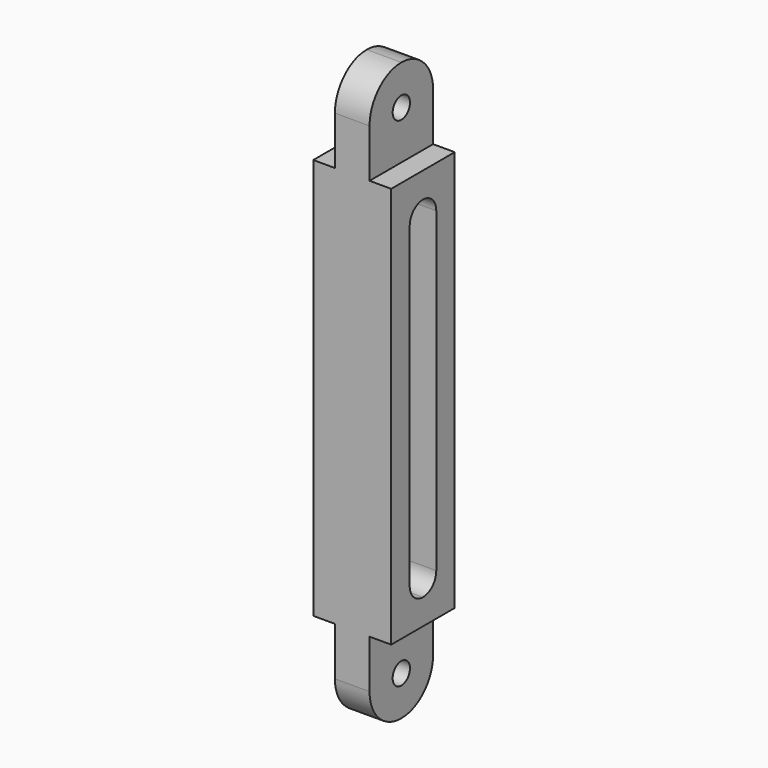
from build123d import *

# Parameters (mm, degrees)
F0_W      = 5.4
F0_H      = 40
F1_DEPTH  = 5.5
F2_W      = 1.5
F2_H      = 6.1
F3_DEPTH  = 5.501
F4_W      = 1.5
F4_H      = 6.1
F5_DEPTH  = 25
F6_W      = 1.5
F6_H      = 6.1
F7_DEPTH  = 5.501
F8_W      = 1.5
F8_H      = 6.1
F9_DEPTH  = 5.501
F10_R     = 2.75
F11_R     = 2.74999
F12_R     = 2.75
F13_R     = 2.74999
F14_W     = 2.3
F14_H     = 24.25
F15_DEPTH = 2.701
F16_DEPTH = 2.701
F17_R     = 1.15
F18_R     = 1.14999
F19_R     = 1.15
F20_R     = 1.14999
F21_R     = 0.75
F22_DEPTH = 3.901
F23_R     = 0.75
F24_DEPTH = 3.901


# Not quite as in the source:
# - a fillet or chamfer is up to 0.001 mm smaller than in the source, because OpenCascade refuses the exact size


with BuildPart() as f1:
    # F0 (on Front) → F1 (new body)
    with BuildSketch(Plane.XZ):
        Rectangle(F0_W, F0_H)
    extrude(amount=F1_DEPTH)

    # F2 (on face) → F3 (cut, through all)
    with BuildSketch(Plane.XZ.offset(5.5)):
        with Locations((-1.95, 16.95)):
            Rectangle(F2_W, F2_H)
    extrude(amount=-F3_DEPTH, mode=Mode.SUBTRACT)

    # F4 (on face) → F5 (cut)
    with BuildSketch(Plane.XZ.offset(5.5)):
        with Locations((1.95, 16.95)):
            Rectangle(F4_W, F4_H)
    extrude(amount=-F5_DEPTH, mode=Mode.SUBTRACT)

    # F6 (on face) → F7 (cut, through all)
    with BuildSketch(Plane.XZ.offset(5.5)):
        with Locations((-1.95, -16.95)):
            Rectangle(F6_W, F6_H)
    extrude(amount=-F7_DEPTH, mode=Mode.SUBTRACT)

    # F8 (on face) → F9 (cut, through all)
    with BuildSketch(Plane.XZ.offset(5.5)):
        with Locations((1.95, -16.95)):
            Rectangle(F8_W, F8_H)
    extrude(amount=-F9_DEPTH, mode=Mode.SUBTRACT)

    # F10
    f10_edges = [f1.edges().sort_by_distance(p)[0] for p in [
        (0, -5.5, 20),
    ]]
    fillet(f10_edges, radius=F10_R)

    # F11 (radius 2.75 in the source; OpenCascade refuses exactly that, so slightly less here)
    f11_edges = [f1.edges().sort_by_distance(p)[0] for p in [
        (0, 0, 20),
    ]]
    fillet(f11_edges, radius=F11_R)

    # F12
    f12_edges = [f1.edges().sort_by_distance(p)[0] for p in [
        (0, 0, -20),
    ]]
    fillet(f12_edges, radius=F12_R)

    # F13 (radius 2.75 in the source; OpenCascade refuses exactly that, so slightly less here)
    f13_edges = [f1.edges().sort_by_distance(p)[0] for p in [
        (0, -5.5, -20),
    ]]
    fillet(f13_edges, radius=F13_R)

    # F14 (on Right) → F15 (cut, through all)
    with BuildSketch(Plane.YZ):
        with Locations((-2.75, 0)):
            Rectangle(F14_W, F14_H)
    extrude(amount=-F15_DEPTH, mode=Mode.SUBTRACT)

    # F14 (on Right) → F16 (cut, through all)
    with BuildSketch(Plane.YZ):
        with Locations((-2.75, 0)):
            Rectangle(F14_W, F14_H)
    extrude(amount=F16_DEPTH, mode=Mode.SUBTRACT)

    # F17
    f17_edges = [f1.edges().sort_by_distance(p)[0] for p in [
        (0, -3.9, 12.125),
    ]]
    fillet(f17_edges, radius=F17_R)

    # F18 (radius 1.15 in the source; OpenCascade refuses exactly that, so slightly less here)
    f18_edges = [f1.edges().sort_by_distance(p)[0] for p in [
        (0, -1.6, 12.125),
    ]]
    fillet(f18_edges, radius=F18_R)

    # F19
    f19_edges = [f1.edges().sort_by_distance(p)[0] for p in [
        (0, -3.9, -12.125),
    ]]
    fillet(f19_edges, radius=F19_R)

    # F20 (radius 1.15 in the source; OpenCascade refuses exactly that, so slightly less here)
    f20_edges = [f1.edges().sort_by_distance(p)[0] for p in [
        (0, -1.6, -12.125),
    ]]
    fillet(f20_edges, radius=F20_R)

    # F21 (on face) → F22 (cut, through all)
    with BuildSketch(Plane.YZ.offset(1.2)):
        with Locations((-2.75, 17.25)):
            Circle(F21_R)
    extrude(amount=-F22_DEPTH, mode=Mode.SUBTRACT)

    # F23 (on face) → F24 (cut, through all)
    with BuildSketch(Plane.YZ.offset(1.2)):
        with Locations((-2.75, -17.25)):
            Circle(F23_R)
    extrude(amount=-F24_DEPTH, mode=Mode.SUBTRACT)


solid = f1.part
